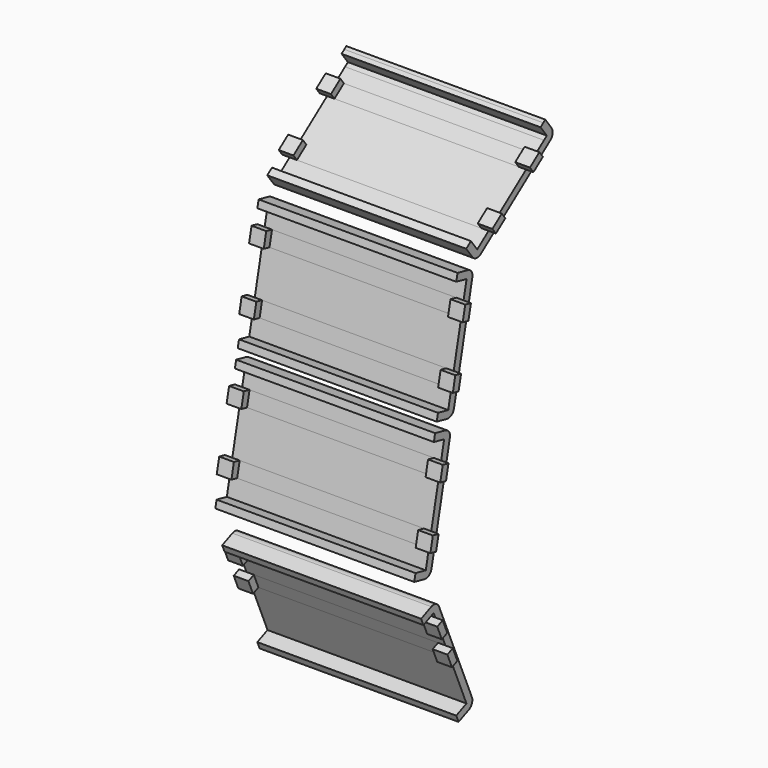
from build123d import *

# Parameters (mm, degrees)
F1_DEPTH = 34.3916
F2_START = 31.8516
F2_DEPTH = 5.08
F3_START = -31.8516
F3_DEPTH = 5.08


with BuildPart() as f1:
    # F0 (on Right) → F1 (new body, symmetric)
    with BuildSketch(Plane.YZ):
        with BuildLine():
            Line((35.5475592049, 135.882533211), (31.1087493632, 136.8430153909))
            Line((31.1087493632, 136.8430153909), (30.5715689534, 134.3604688743))
            Line((30.5715689534, 134.3604688743), (35.010378795, 133.3999866944))
            Line((35.010378795, 133.3999866944), (33.7174203827, 127.4246582133))
            Line((33.7174203827, 127.4246582133), (32.643059563, 122.45956518))
            Line((32.643059563, 122.45956518), (29.4417548033, 107.6649303911))
            Line((29.4417548033, 107.6649303911), (28.3673939836, 102.6998373579))
            Line((28.3673939836, 102.6998373579), (27.077006821, 96.7363917505))
            Line((27.077006821, 96.7363917505), (22.6381969794, 97.6968739305))
            Line((22.6381969794, 97.6968739305), (22.1010165695, 95.2143274138))
            Line((22.1010165695, 95.2143274138), (26.5398264112, 94.2538452339))
            ThreePointArc((26.5398264112, 94.2538452339), (28.452588387, 94.6011223635), (29.5595533377, 96.1992113407))
            Line((29.5595533377, 96.1992113407), (37.4929253116, 132.8628062845))
            ThreePointArc((37.4929253116, 132.8628062845), (37.1456481821, 134.7755682604), (35.5475592049, 135.882533211))
        make_face()
    extrude(amount=F1_DEPTH, both=True)

    # F0 (on Right) → F2, piece 2 (join)
    with BuildSketch(Plane.YZ.offset(F2_START)):
        Polygon((32.643059563, 122.45956518), (33.7174203827, 127.4246582133), (31.2348738661, 127.9618386231), (30.1605130463, 122.9967455899), align=None)
        Polygon((25.884847467, 103.2370177677), (28.3673939836, 102.6998373579), (29.4417548033, 107.6649303911), (26.9592082867, 108.202110801), align=None)
    extrude(amount=F2_DEPTH)

    # F0 (on Right) → F3, piece 2 (join)
    with BuildSketch(Plane.YZ.offset(F3_START)):
        Polygon((32.643059563, 122.45956518), (33.7174203827, 127.4246582133), (31.2348738661, 127.9618386231), (30.1605130463, 122.9967455899), align=None)
        Polygon((25.884847467, 103.2370177677), (28.3673939836, 102.6998373579), (29.4417548033, 107.6649303911), (26.9592082867, 108.202110801), align=None)
    extrude(amount=-F3_DEPTH)


with BuildPart() as f1b:
    # F0 (on Right) → F1, piece 2 (new body, symmetric)
    with BuildSketch(Plane.YZ):
        with BuildLine():
            Line((12.9357939022, 52.8578095868), (12.3986134924, 50.3752630702))
            Line((12.3986134924, 50.3752630702), (16.837423334, 49.4147808903))
            ThreePointArc((16.837423334, 49.4147808903), (18.7501853099, 49.7620580199), (19.8571502605, 51.3601469971))
            Line((19.8571502605, 51.3601469971), (27.7905222345, 88.0237419409))
            ThreePointArc((27.7905222345, 88.0237419409), (27.4432451049, 89.9365039168), (25.8451561277, 91.0434688674))
            Line((25.8451561277, 91.0434688674), (21.4063462861, 92.0039510473))
            Line((21.4063462861, 92.0039510473), (20.8691658762, 89.5214045307))
            Line((20.8691658762, 89.5214045307), (25.3079757178, 88.5609223508))
            Line((25.3079757178, 88.5609223508), (24.0175885553, 82.5974767434))
            Line((24.0175885553, 82.5974767434), (22.9432277355, 77.6323837102))
            Line((22.9432277355, 77.6323837102), (19.7419229759, 62.8377489213))
            Line((19.7419229759, 62.8377489213), (18.6675621562, 57.872655888))
            Line((18.6675621562, 57.872655888), (17.3746037439, 51.8973274069))
            Line((17.3746037439, 51.8973274069), (12.9357939022, 52.8578095868))
        make_face()
    extrude(amount=F1_DEPTH, both=True)

    # F0 (on Right) → F2, piece 3 (join)
    with BuildSketch(Plane.YZ.offset(F2_START)):
        Polygon((16.1850156395, 58.4098362979), (18.6675621562, 57.872655888), (19.7419229759, 62.8377489213), (17.2593764593, 63.3749293312), align=None)
        Polygon((22.9432277355, 77.6323837102), (24.0175885553, 82.5974767434), (21.5350420386, 83.1346571533), (20.4606812189, 78.16956412), align=None)
    extrude(amount=F2_DEPTH)

    # F0 (on Right) → F3, piece 3 (join)
    with BuildSketch(Plane.YZ.offset(F3_START)):
        Polygon((22.9432277355, 77.6323837102), (24.0175885553, 82.5974767434), (21.5350420386, 83.1346571533), (20.4606812189, 78.16956412), align=None)
        Polygon((16.1850156395, 58.4098362979), (18.6675621562, 57.872655888), (19.7419229759, 62.8377489213), (17.2593764593, 63.3749293312), align=None)
    extrude(amount=-F3_DEPTH)


with BuildPart() as f1c:
    # F0 (on Right) → F1, piece 3 (new body, symmetric)
    with BuildSketch(Plane.YZ):
        with BuildLine():
            Line((30.5493542935, 2.3257501254), (31.5401391658, 0))
            Line((31.5401391658, 0), (31.5707651968, 0))
            Line((31.5707651968, 0), (35.9613821509, 1.8704317419))
            ThreePointArc((35.9613821509, 1.8704317419), (37.3221722578, 3.2587797047), (37.302685911, 5.2027138762))
            Line((37.302685911, 5.2027138762), (23.1128714591, 38.5116224639))
            ThreePointArc((23.1128714591, 38.5116224639), (21.7245234962, 39.8724125708), (19.7805893247, 39.852926224))
            Line((19.7805893247, 39.852926224), (15.3640506544, 37.9714516603))
            Line((15.3640506544, 37.9714516603), (16.3595398415, 35.6346587131))
            Line((16.3595398415, 35.6346587131), (20.7760785118, 37.5161332768))
            Line((20.7760785118, 37.5161332768), (21.4843682503, 35.8535070154))
            Line((21.4843682503, 35.8535070154), (23.4753466245, 31.1799211209))
            Line((23.4753466245, 31.1799211209), (25.8665425285, 25.5668719827))
            Line((25.8665425285, 25.5668719827), (27.8575209028, 20.8932860882))
            Line((27.8575209028, 20.8932860882), (34.9658929638, 4.2072246891))
            Line((34.9658929638, 4.2072246891), (30.5493542935, 2.3257501254))
        make_face()
    extrude(amount=F1_DEPTH, both=True)

    # F0 (on Right) → F2, piece 4 (join)
    with BuildSketch(Plane.YZ.offset(F2_START)):
        Polygon((21.1385536773, 30.1844319338), (23.4753466245, 31.1799211209), (21.4843682503, 35.8535070154), (19.147575303, 34.8580178283), align=None)
        Polygon((25.5207279555, 19.8977969011), (27.8575209028, 20.8932860882), (25.8665425285, 25.5668719827), (23.5297495813, 24.5713827956), align=None)
    extrude(amount=F2_DEPTH)

    # F0 (on Right) → F3, piece 4 (join)
    with BuildSketch(Plane.YZ.offset(F3_START)):
        Polygon((25.5207279555, 19.8977969011), (27.8575209028, 20.8932860882), (25.8665425285, 25.5668719827), (23.5297495813, 24.5713827956), align=None)
        Polygon((21.1385536773, 30.1844319338), (23.4753466245, 31.1799211209), (21.4843682503, 35.8535070154), (19.147575303, 34.8580178283), align=None)
    extrude(amount=-F3_DEPTH)


with BuildPart() as f1d:
    # F0 (on Right) → F1, piece 4 (new body, symmetric)
    with BuildSketch(Plane.YZ):
        with BuildLine():
            ThreePointArc((70.6874244764, 164.5491375), (70.0510915867, 162.8675752701), (68.4609272063, 162.0285589874))
            Line((68.4609272063, 162.0285589874), (64.7923923036, 159.296159841))
            Line((64.7923923036, 159.296159841), (60.7182854085, 156.2616824549))
            Line((60.7182854085, 156.2616824549), (48.5785484084, 147.2197602993))
            Line((48.5785484084, 147.2197602993), (44.5044415132, 144.1852829132))
            Line((44.5044415132, 144.1852829132), (39.6013859607, 140.5333877666))
            Line((39.6013859607, 140.5333877666), (36.8885529895, 144.1756530093))
            Line((36.8885529895, 144.1756530093), (34.8514995419, 142.6584143163))
            Line((34.8514995419, 142.6584143163), (37.5643325131, 139.0161490735))
            ThreePointArc((37.5643325131, 139.0161490735), (39.2338214228, 138.0201236916), (41.1186246537, 138.496334319))
            Line((41.1186246537, 138.496334319), (71.2029360576, 160.9037391763))
            ThreePointArc((71.2029360576, 160.9037391763), (72.1989614395, 162.573228086), (71.7227508122, 164.4580313169))
            Line((71.7227508122, 164.4580313169), (70.6874244764, 165.8480664454))
            Line((70.6874244764, 165.8480664454), (70.6874244764, 164.5491375))
        make_face()
        with BuildLine():
            Line((69.6856973646, 162.9407926238), (68.4609272063, 162.0285589874))
            ThreePointArc((68.4609272063, 162.0285589874), (70.0510915867, 162.8675752701), (70.6874244764, 164.5491375))
            Line((70.6874244764, 164.5491375), (70.6874244764, 165.8480664454))
            Line((70.6874244764, 165.8480664454), (69.009917841, 168.1002965597))
            Line((69.009917841, 168.1002965597), (68.1474244764, 167.4578940214))
            Line((68.1474244764, 167.4578940214), (68.1474244764, 165.0060867035))
            Line((68.1474244764, 165.0060867035), (69.6856973646, 162.9407926238))
        make_face()
        Polygon((68.1474244764, 165.0060867035), (68.1474244764, 167.4578940214), (66.9728643934, 166.5830578666), align=None)
    extrude(amount=F1_DEPTH, both=True)

    # F0 (on Right) → F2 (join)
    with BuildSketch(Plane.YZ.offset(F2_START)):
        Polygon((60.7182854085, 156.2616824549), (64.7923923036, 159.296159841), (63.2751536106, 161.3332132886), (59.2010467154, 158.2987359025), align=None)
        Polygon((44.5044415132, 144.1852829132), (48.5785484084, 147.2197602993), (47.0613097153, 149.2568137468), (42.9872028202, 146.2223363607), align=None)
    extrude(amount=F2_DEPTH)

    # F0 (on Right) → F3 (join)
    with BuildSketch(Plane.YZ.offset(F3_START)):
        Polygon((60.7182854085, 156.2616824549), (64.7923923036, 159.296159841), (63.2751536106, 161.3332132886), (59.2010467154, 158.2987359025), align=None)
        Polygon((44.5044415132, 144.1852829132), (48.5785484084, 147.2197602993), (47.0613097153, 149.2568137468), (42.9872028202, 146.2223363607), align=None)
    extrude(amount=-F3_DEPTH)


solid = Compound([f1.part, f1b.part, f1c.part, f1d.part])
